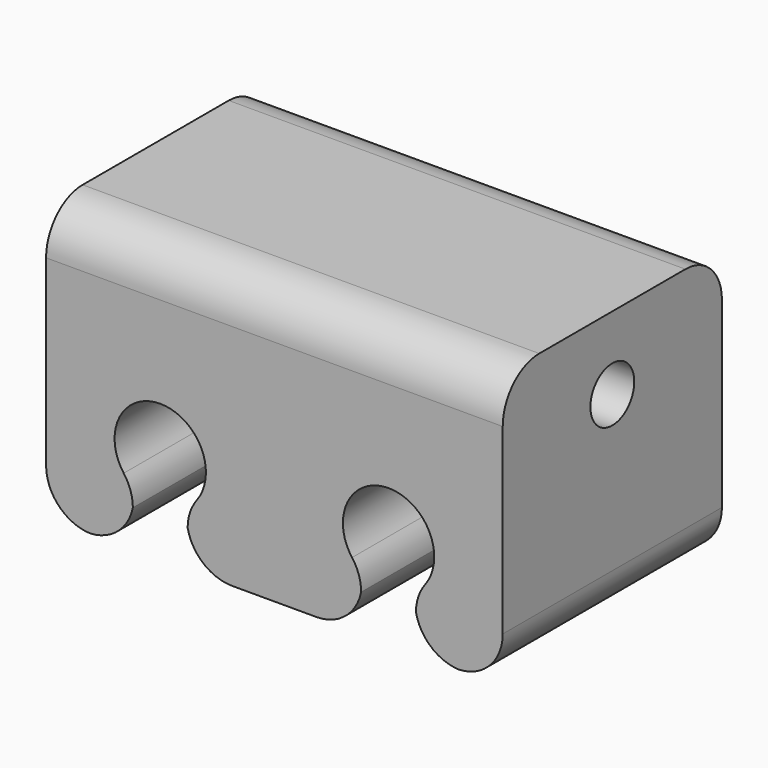
from build123d import *

# Parameters (mm, degrees)
F1_DEPTH    = 30
F2_R        = 5
F3_T1_DEPTH = 54.4948974279
F3_T3_DEPTH = 55
F4_R        = 5
F6_D        = 6


# Not quite as in the source:
# - a fillet or chamfer that OpenCascade refuses, or shapes differently, is made with other operations: its cross-section is extruded or revolved along the edge and cut away or added


with BuildPart() as f1:
    # F0 (on Front) → F1 (new body)
    with BuildSketch(Plane.XZ):
        with BuildLine():
            Line((0, 30), (0, 0))
            Line((0, 0), (9.5, 0))
            Line((9.5, 0), (9.5, 6))
            ThreePointArc((9.5, 6), (10.2639320225, 14.472135955), (17.5, 10))
            ThreePointArc((17.5, 10), (16.972135955, 7.7639320225), (15.5, 6))
            Line((15.5, 6), (15.5, 0))
            Line((15.5, 0), (34.5, 0))
            Line((34.5, 0), (34.5, 6))
            ThreePointArc((34.5, 6), (35.2639320225, 14.472135955), (42.5, 10))
            ThreePointArc((42.5, 10), (41.972135955, 7.7639320225), (40.5, 6))
            Line((40.5, 6), (40.5, 0))
            Line((40.5, 0), (50, 0))
            Line((50, 0), (50, 30))
            Line((50, 30), (0, 30))
        make_face()
    extrude(amount=F1_DEPTH)

    # F2
    f2_edges = [f1.edges().sort_by_distance(p)[0] for p in [
        (40.5, -15, 6),
        (34.5, -15, 6),
        (9.5, -15, 6),
        (15.5, -15, 6),
    ]]
    fillet(f2_edges, radius=F2_R)

    # F3: fillet of radius 5 on 6 edges, made by hand

    # F3_s2 → F3_t1 (cut)
    with BuildSketch(Plane.XZ.offset(-12.2474487139)):
        with BuildLine():
            ThreePointArc((4.6010205144, 0), (7.7632981746, 1.1270166538), (9.5, 4))
            Line((9.5, 4), (9.5, 0))
            Line((9.5, 0), (4.6010205144, 0))
        make_face()
        with BuildLine():
            ThreePointArc((34.5, 4), (32.7632981746, 1.1270166538), (29.6010205144, 0))
            Line((29.6010205144, 0), (34.5, 0))
            Line((34.5, 0), (34.5, 4))
        make_face()
        with BuildLine():
            ThreePointArc((40.5, 4), (42.2367018254, 1.1270166538), (45.3989794856, 0))
            Line((45.3989794856, 0), (40.5, 0))
            Line((40.5, 0), (40.5, 4))
        make_face()
        with BuildLine():
            ThreePointArc((20.3989794856, 0), (17.2367018254, 1.1270166538), (15.5, 4))
            Line((15.5, 4), (15.5, 0))
            Line((15.5, 0), (20.3989794856, 0))
        make_face()
    extrude(amount=F3_T1_DEPTH, mode=Mode.SUBTRACT)

    # F3_s4 → F3_t3 (cut)
    with BuildSketch(Plane.XZ.offset(-12.5)):
        with BuildLine():
            ThreePointArc((45, 0), (48.5355339059, 1.4644660941), (50, 5))
            Line((50, 5), (50, 0))
            Line((50, 0), (45, 0))
        make_face()
        with BuildLine():
            ThreePointArc((0, 5), (1.4644660941, 1.4644660941), (5, 0))
            Line((5, 0), (0, 0))
            Line((0, 0), (0, 5))
        make_face()
    extrude(amount=F3_T3_DEPTH, mode=Mode.SUBTRACT)

    # F4
    f4_edges = [f1.edges().sort_by_distance(p)[0] for p in [
        (25, -30, 30),
        (25, 0, 30),
    ]]
    fillet(f4_edges, radius=F4_R)

    # F6 (through all)
    with Locations(Plane.YZ.offset(50)):
        with Locations((-15, 22)):
            Hole(F6_D / 2)


solid = f1.part
